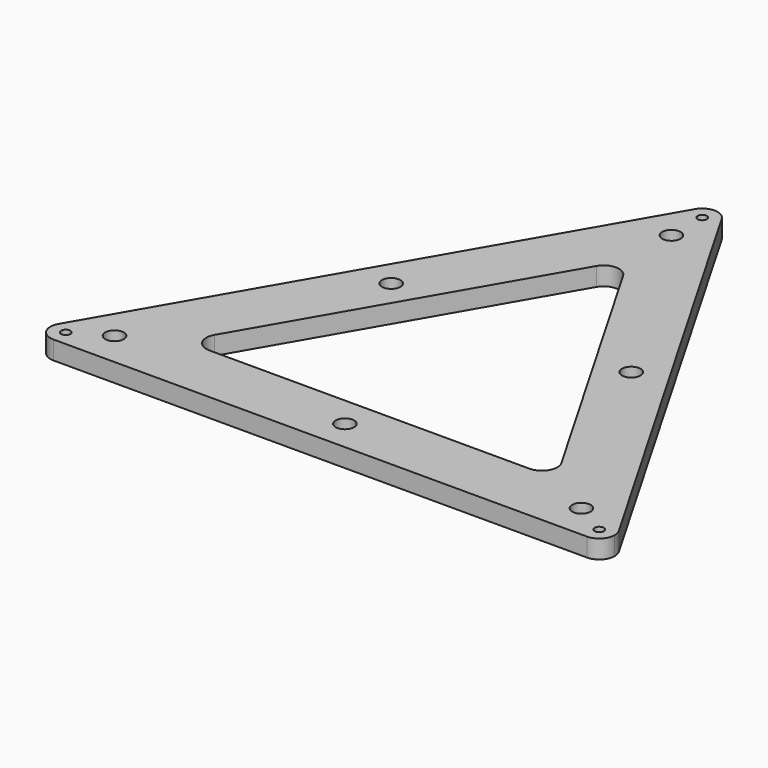
from build123d import *

# Parameters (mm, degrees)
F1_R            = 3
F1_R_2          = 1.5
F2_DEPTH        = 6
F3_R            = 5
F4_R            = 3
F5_DEPTH        = 12.5
F5_COPIES_COUNT = 3


# Not quite as in the source:
# - a pattern or mirror of a feature is missing from the dataset's text; its kind, count and spacing are read off the source's solid


with BuildPart() as f2:
    # F1 (on Top) → F2 (new body)
    with BuildSketch(Plane.XY):
        with BuildLine():
            ThreePointArc((4.3301270189, 102.5), (4.8296291314, 101.2940952255), (5, 100))
            ThreePointArc((5, 100), (-1.2940952255, 95.1703708686), (-4.3301270189, 102.5))
            Line((-4.3301270189, 102.5), (-90.9326673974, -47.5))
            ThreePointArc((-90.9326673974, -47.5), (-85.3084451529, -45.1703708686), (-81.6025403784, -50))
            ThreePointArc((-81.6025403784, -50), (-83.0670064725, -53.5355339059), (-86.6025403784, -55))
            Line((-86.6025403784, -55), (86.6025403784, -55))
            ThreePointArc((86.6025403784, -55), (82.2724133595, -47.5), (90.9326673974, -47.5))
            Line((90.9326673974, -47.5), (4.3301270189, 102.5))
        make_face()
        with Locations((-38.9711431703, 22.5)):
            Circle(F1_R, mode=Mode.SUBTRACT)
        with Locations((0, -45)):
            Circle(F1_R, mode=Mode.SUBTRACT)
        Polygon((60.6217782649, -35), (-60.6217782649, -35), (0, 70), align=None, mode=Mode.SUBTRACT)
        with Locations((38.9711431703, 22.5)):
            Circle(F1_R, mode=Mode.SUBTRACT)
        with BuildLine():
            ThreePointArc((91.6025403784, -50), (91.4321695099, -48.7059047745), (90.9326673974, -47.5))
            ThreePointArc((90.9326673974, -47.5), (82.2724133595, -47.5), (86.6025403784, -55))
            ThreePointArc((86.6025403784, -55), (90.1380742844, -53.5355339059), (91.6025403784, -50))
        make_face()
        with Locations((86.6025403784, -50)):
            Circle(F1_R_2, mode=Mode.SUBTRACT)
        with BuildLine():
            ThreePointArc((-81.6025403784, -50), (-85.3084451529, -45.1703708686), (-90.9326673974, -47.5))
            ThreePointArc((-90.9326673974, -47.5), (-90.9326673974, -52.5), (-86.6025403784, -55))
            ThreePointArc((-86.6025403784, -55), (-83.0670064725, -53.5355339059), (-81.6025403784, -50))
        make_face()
        with Locations((-86.6025403784, -50)):
            Circle(F1_R_2, mode=Mode.SUBTRACT)
        with BuildLine():
            ThreePointArc((-4.3301270189, 102.5), (-1.2940952255, 95.1703708686), (5, 100))
            ThreePointArc((5, 100), (4.8296291314, 101.2940952255), (4.3301270189, 102.5))
            ThreePointArc((4.3301270189, 102.5), (0, 105), (-4.3301270189, 102.5))
        make_face()
        with Locations((0, 100)):
            Circle(F1_R_2, mode=Mode.SUBTRACT)
    extrude(amount=F2_DEPTH)

    # F3
    f3_edges = [f2.edges().sort_by_distance(p)[0] for p in [
        (0, 70, 3),
        (-60.621778, -35, 3),
        (60.621778, -35, 3),
    ]]
    fillet(f3_edges, radius=F3_R)

    # F4 (on Top) → F5 (cut, symmetric)
    with BuildSketch(Plane.XY):
        with Locations((0, 87.5)):
            Circle(F4_R)
    f5 = extrude(amount=F5_DEPTH, both=True, mode=Mode.SUBTRACT)

    # F5_copies: F5 ×3 about axis
    f5_copies_axis = Axis((0, 0, 0), (0, 0, 1))
    for i in range(1, F5_COPIES_COUNT):
        add(f5.rotate(f5_copies_axis, i * 360 / F5_COPIES_COUNT), mode=Mode.SUBTRACT)


solid = f2.part
